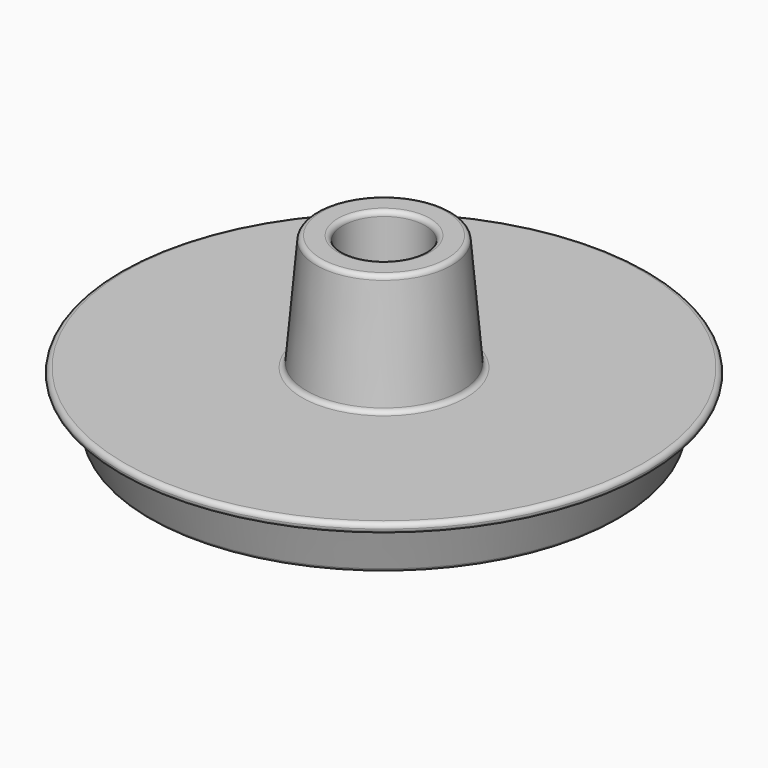
from build123d import *

# Parameters (mm, degrees)
F0_R     = 27.25
F0_R_2   = 25.75
F0_R_3   = 24.25
F1_DEPTH = 1
F2_DEPTH = 5
F2_TAPER = 17.5
F3_R     = 8
F4_DEPTH = 12
F4_TAPER = 5
F5_R     = 4.25
F6_DEPTH = 18
F7_R     = 0.49999


# Not quite as in the source:
# - a fillet or chamfer is up to 0.001 mm smaller than in the source, because OpenCascade refuses the exact size


with BuildPart() as f1:
    # F0 (on Top) → F1 (new body)
    with BuildSketch(Plane.XY):
        Circle(F0_R)
        Circle(F0_R_2, mode=Mode.SUBTRACT)
        Circle(F0_R_2)
        Circle(F0_R_3, mode=Mode.SUBTRACT)
        Circle(F0_R_3)
    extrude(amount=F1_DEPTH)

    # F0 (on Top) → F2 (join)
    with BuildSketch(Plane.XY):
        Circle(F0_R_2)
        Circle(F0_R_3, mode=Mode.SUBTRACT)
        Circle(F0_R_3)
    extrude(amount=-F2_DEPTH, taper=F2_TAPER)

    # F3 (on face) → F4 (join)
    with BuildSketch(Plane.XY.offset(1)):
        Circle(F3_R)
    extrude(amount=F4_DEPTH, taper=F4_TAPER)

    # F5 (on face) → F6 (cut, through all)
    with BuildSketch(Plane.XY.offset(13)):
        Circle(F5_R)
    extrude(amount=-F6_DEPTH, mode=Mode.SUBTRACT)

    # F7 (radius 0.5 in the source; OpenCascade refuses exactly that, so slightly less here)
    f7_edges = [f1.edges().sort_by_distance(p)[0] for p in [
        (-24.173506, 0, -5),
        (-27.25, 0, 0),
        (-27.25, 0, 1),
        (-4.25, 0, -5),
        (-8, 0, 1),
        (-6.950136, 0, 13),
        (-4.25, 0, 13),
    ]]
    fillet(f7_edges, radius=F7_R)


solid = f1.part
